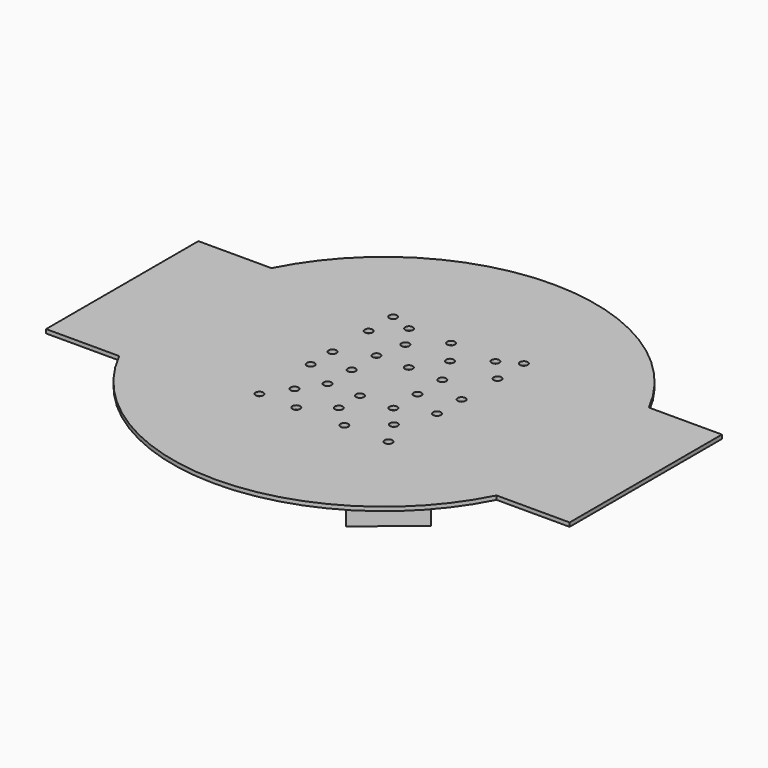
from build123d import *

# Parameters (mm, degrees)
F1_DEPTH = 2.5
F2_DEPTH = 20
F3_D     = 5
F3_DEPTH = 200
F3_TIP   = 1.5021515476


# Not quite as in the source:
# - a feature names something its author has since deleted; it is built from what else it names


with BuildPart() as f1:
    # F0 (on Top) → F1 (new body)
    with BuildSketch(Plane.XY):
        with BuildLine():
            ThreePointArc((120.5299497215, -60.8073286712), (131.3326753181, -31.252654188), (135, 0))
            ThreePointArc((135, 0), (131.3326753181, 31.252654188), (120.5299497215, 60.8073286712))
            ThreePointArc((120.5299497215, 60.8073286712), (0, 135), (-120.5299497215, 60.8073286712))
            ThreePointArc((-120.5299497215, 60.8073286712), (-135, 0), (-120.5299497215, -60.8073286712))
            ThreePointArc((-120.5299497215, -60.8073286712), (0, -135), (120.5299497215, -60.8073286712))
        make_face()
        Polygon((88.5368213058, -73.284752667), (55.893484503, -100.0614613295), (46.9403453171, -59.9641390145), align=None, mode=Mode.SUBTRACT)
        Polygon((-117.2483563423, -17.961492762), (-117.2483563423, 31.1308540404), (-85.331723094, 0), align=None, mode=Mode.SUBTRACT)
        Polygon((58.2080259919, 55.2336238325), (72.7635622025, 97.6980701089), (103.1368598342, 61.4694543183), align=None, mode=Mode.SUBTRACT)
        with BuildLine():
            ThreePointArc((-120.5299497215, -60.8073286712), (-135, 0), (-120.5299497215, 60.8073286712))
            Line((-120.5299497215, 60.8073286712), (-167.2347635031, 60.8073286712))
            Line((-167.2347635031, 60.8073286712), (-167.2347635031, -60.8073286712))
            Line((-167.2347635031, -60.8073286712), (-120.5299497215, -60.8073286712))
        make_face()
        with BuildLine():
            ThreePointArc((120.5299497215, 60.8073286712), (131.3326753181, 31.252654188), (135, 0))
            ThreePointArc((135, 0), (131.3326753181, -31.252654188), (120.5299497215, -60.8073286712))
            Line((120.5299497215, -60.8073286712), (167.2347635031, -60.8073286712))
            Line((167.2347635031, -60.8073286712), (167.2347635031, 60.8073286712))
            Line((167.2347635031, 60.8073286712), (120.5299497215, 60.8073286712))
        make_face()
        Polygon((-85.331723094, 0), (-117.2483563423, 31.1308540404), (-117.2483563423, -17.961492762), align=None)
        Polygon((103.1368598342, 61.4694543183), (72.7635622025, 97.6980701089), (58.2080259919, 55.2336238325), align=None)
        Polygon((46.9403453171, -59.9641390145), (55.893484503, -100.0614613295), (88.5368213058, -73.284752667), align=None)
    extrude(amount=F1_DEPTH)

    # F0 (on Top) → F2 (join)
    with BuildSketch(Plane.XY):
        Polygon((-85.331723094, 0), (-117.2483563423, 31.1308540404), (-117.2483563423, -17.961492762), align=None)
        Polygon((103.1368598342, 61.4694543183), (72.7635622025, 97.6980701089), (58.2080259919, 55.2336238325), align=None)
        Polygon((46.9403453171, -59.9641390145), (55.893484503, -100.0614613295), (88.5368213058, -73.284752667), align=None)
    extrude(amount=-F2_DEPTH)

    # F3
    with Locations(Plane(origin=(0, 0, 0), x_dir=(1, 0, 0), z_dir=(0, 0, -1))):
        with Locations((-40.2909182012, -57.7073432505), (-40.2909182012, -38.0536355078), (-40.2909182012, -9.2816902325), (-40.2909182012, 8.147473447), (-40.2909182012, 49.0921735764), (-30.054744333, 33.8762365282), (-16.7753826827, 49.0921735764), (-20.6485316157, 19.2136075348), (-20.6485316157, 0), (-20.6485316157, -19.7945162654), (-16.7753826827, -38.0536355078), (-26.1815954, -52.7162663639), (0, -53.5462275147), (11.7199122906, -38.0536355078), (0, -19.7945162654), (0, 19.2136075348), (0, 36.0894650221), (13.9331379905, 49.0921735764), (42.1517826617, 49.0921735764), (32.7455736697, 33.0462753773), (21.4027836919, 19.2136075348), (21.4027836919, 0), (21.4027836919, -19.7945162654), (29.7023877501, -51.8863089383), (42.1517826617, -58.9785054326), (42.1517826617, -38.0536355078), (42.1517826617, -9.2816902325), (42.1517826617, 10.3607000783)):
            Hole(F3_D / 2, depth=F3_DEPTH)
            with Locations((0, 0, -(F3_DEPTH + F3_TIP / 2))):  # 118° drill point
                Cone(0, F3_D / 2, F3_TIP, mode=Mode.SUBTRACT)


solid = f1.part
